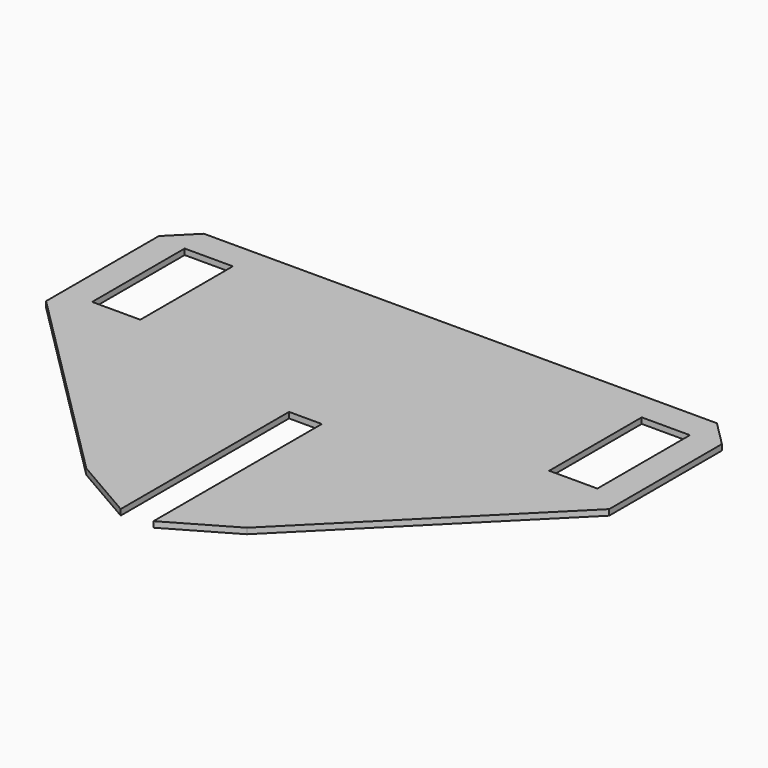
from build123d import *

# Parameters (mm, degrees)
F0_W     = 25
F0_H     = 60
F1_DEPTH = 3


# Not quite as in the source:
# - a feature names something its author has since deleted; it is built from what else it names


with BuildPart() as f1:
    # F0 (on Top) → F1 (new body)
    with BuildSketch(Plane.XY):
        Polygon((132.6056759823, 80.5817515949), (-133.4943240177, 80.5817515949), (-146.4943240177, 67.5817515949), (-146.4943240177, -5.5212787854), (-42.0973543981, -109.9182484051), (-8.9443240177, -129.0591594196), (-8.9443240177, -19.9182484051), (8.0556759823, -19.9182484051), (8.0556759823, -129.0591594196), (41.2087063626, -109.9182484051), (145.6056759823, -5.5212787854), (145.6056759823, 67.5817515949), align=None)
        with Locations((-118.9943240177, 35.5817515949)):
            Rectangle(F0_W, F0_H, mode=Mode.SUBTRACT)
        with Locations((118.1056759823, 35.5817515949)):
            Rectangle(F0_W, F0_H, mode=Mode.SUBTRACT)
    extrude(amount=F1_DEPTH)


solid = f1.part
